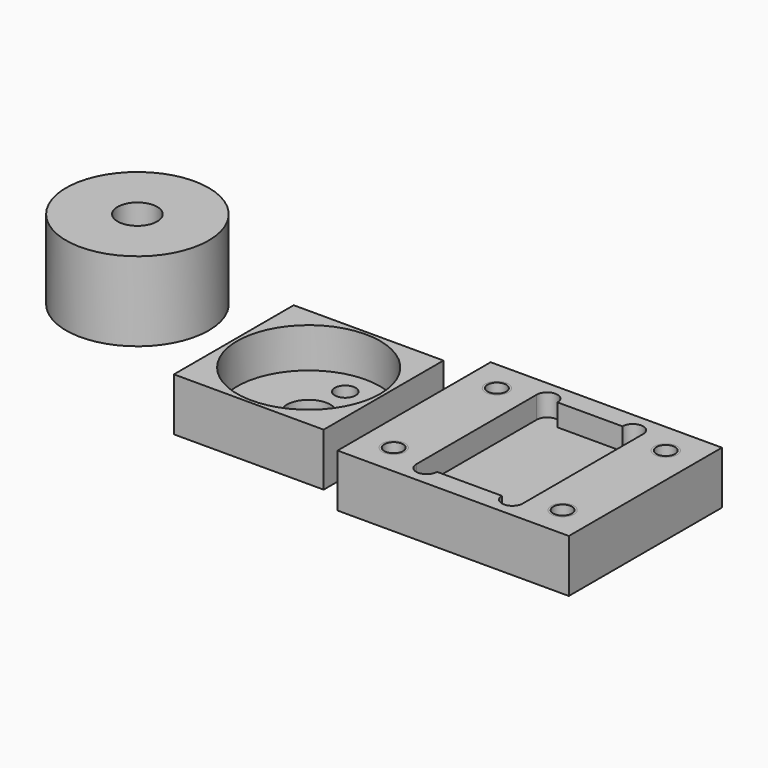
from build123d import *

# Parameters (mm, degrees)
F0_W     = 36
F0_H     = 36
F0_R     = 2.5
F1_DEPTH = 12.7
F2_DEPTH = 9.585
F3_W     = 55.6
F3_H     = 46
F3_R     = 2.75
F3_R_2   = 2.25
F4_DEPTH = 12.7
F5_DEPTH = 11.7
F6_R     = 17.145
F6_R_2   = 4.7625
F7_DEPTH = 19.05
F8_DEPTH = 12.7
F9_DEPTH = 5.3


# Not quite as in the source:
# - a length typed as a fraction of an inch, garbled in the dataset ("3 / 203.2 mm" for 3/8 in), is restored


with BuildPart() as f1:
    # F0 (on Top) → F1 (new body)
    with BuildSketch(Plane.XY):
        Rectangle(F0_W, F0_H)
        with BuildLine():
            ThreePointArc((-17.2, 0), (0, 17.2), (17.2, 0))
            ThreePointArc((17.2, 0), (0, -17.2), (-17.2, 0))
        make_face(mode=Mode.SUBTRACT)
        with BuildLine():
            ThreePointArc((-17.2, 0), (0, -17.2), (17.2, 0))
            ThreePointArc((17.2, 0), (0, 17.2), (-17.2, 0))
        make_face()
        with Locations((0, -10.98125)):
            Circle(F0_R, mode=Mode.SUBTRACT)
        with BuildLine():
            ThreePointArc((5.2625, 0), (0, -5.2625), (-5.2625, 0))
            ThreePointArc((-5.2625, 0), (0, 5.2625), (5.2625, 0))
        make_face(mode=Mode.SUBTRACT)
        with Locations((0, 10.98125)):
            Circle(F0_R, mode=Mode.SUBTRACT)
    extrude(amount=-F1_DEPTH)

    # F0 (on Top) → F2 (cut)
    with BuildSketch(Plane.XY):
        with BuildLine():
            ThreePointArc((-17.2, 0), (0, -17.2), (17.2, 0))
            ThreePointArc((17.2, 0), (0, 17.2), (-17.2, 0))
        make_face()
        with Locations((0, -10.98125)):
            Circle(F0_R, mode=Mode.SUBTRACT)
        with BuildLine():
            ThreePointArc((5.2625, 0), (0, -5.2625), (-5.2625, 0))
            ThreePointArc((-5.2625, 0), (0, 5.2625), (5.2625, 0))
        make_face(mode=Mode.SUBTRACT)
        with Locations((0, 10.98125)):
            Circle(F0_R, mode=Mode.SUBTRACT)
    extrude(amount=-F2_DEPTH, mode=Mode.SUBTRACT)


with BuildPart() as f4:
    # F3 (on Top) → F4 (new body)
    with BuildSketch(Plane.XY):
        with Locations((53.1422479868, 0)):
            Rectangle(F3_W, F3_H)
        with Locations((32.8422479868, -15.5)):
            Circle(F3_R, mode=Mode.SUBTRACT)
        with Locations((73.4422479868, -15.5)):
            Circle(F3_R, mode=Mode.SUBTRACT)
        with BuildLine():
            Line((40.3422479868, -18.1), (40.3422479868, 18.1))
            ThreePointArc((40.3422479868, 18.1), (42.8422479868, 20.6), (45.3422479868, 18.1))
            Line((45.3422479868, 18.1), (60.9422479868, 18.1))
            ThreePointArc((60.9422479868, 18.1), (63.4422479868, 20.6), (65.9422479868, 18.1))
            Line((65.9422479868, 18.1), (65.9422479868, -18.1))
            ThreePointArc((65.9422479868, -18.1), (63.4422479868, -20.6), (60.9422479868, -18.1))
            Line((60.9422479868, -18.1), (45.3422479868, -18.1))
            ThreePointArc((45.3422479868, -18.1), (42.8422479868, -20.6), (40.3422479868, -18.1))
        make_face(mode=Mode.SUBTRACT)
        with Locations((32.8422479868, 15.5)):
            Circle(F3_R, mode=Mode.SUBTRACT)
        with Locations((73.4422479868, 15.5)):
            Circle(F3_R, mode=Mode.SUBTRACT)
        with BuildLine():
            ThreePointArc((45.3422479868, 18.1), (42.8422479868, 20.6), (40.3422479868, 18.1))
            Line((40.3422479868, 18.1), (40.3422479868, -18.1))
            ThreePointArc((40.3422479868, -18.1), (42.8422479868, -20.6), (45.3422479868, -18.1))
            Line((45.3422479868, -18.1), (60.9422479868, -18.1))
            ThreePointArc((60.9422479868, -18.1), (63.4422479868, -20.6), (65.9422479868, -18.1))
            Line((65.9422479868, -18.1), (65.9422479868, 18.1))
            ThreePointArc((65.9422479868, 18.1), (63.4422479868, 20.6), (60.9422479868, 18.1))
            Line((60.9422479868, 18.1), (45.3422479868, 18.1))
        make_face()
        with Locations((32.8422479868, 15.5)):
            Circle(F3_R)
        with Locations((32.8422479868, 15.5)):
            Circle(F3_R_2, mode=Mode.SUBTRACT)
        with Locations((32.8422479868, -15.5)):
            Circle(F3_R)
        with Locations((32.8422479868, -15.5)):
            Circle(F3_R_2, mode=Mode.SUBTRACT)
        with Locations((73.4422479868, -15.5)):
            Circle(F3_R)
        with Locations((73.4422479868, -15.5)):
            Circle(F3_R_2, mode=Mode.SUBTRACT)
        with Locations((73.4422479868, 15.5)):
            Circle(F3_R)
        with Locations((73.4422479868, 15.5)):
            Circle(F3_R_2, mode=Mode.SUBTRACT)
    extrude(amount=-F4_DEPTH)

    # F3 (on Top) → F5 (cut)
    with BuildSketch(Plane.XY):
        with BuildLine():
            ThreePointArc((45.3422479868, 18.1), (42.8422479868, 20.6), (40.3422479868, 18.1))
            Line((40.3422479868, 18.1), (40.3422479868, -18.1))
            ThreePointArc((40.3422479868, -18.1), (42.8422479868, -20.6), (45.3422479868, -18.1))
            Line((45.3422479868, -18.1), (60.9422479868, -18.1))
            ThreePointArc((60.9422479868, -18.1), (63.4422479868, -20.6), (65.9422479868, -18.1))
            Line((65.9422479868, -18.1), (65.9422479868, 18.1))
            ThreePointArc((65.9422479868, 18.1), (63.4422479868, 20.6), (60.9422479868, 18.1))
            Line((60.9422479868, 18.1), (45.3422479868, 18.1))
        make_face()
    extrude(amount=-F5_DEPTH, mode=Mode.SUBTRACT)


with BuildPart() as f7:
    # F6 (on Top) → F7 (new body)
    with BuildSketch(Plane.XY):
        with Locations((-41.1721505225, 0)):
            Circle(F6_R)
        with Locations((-41.1721505225, 0)):
            Circle(F6_R_2, mode=Mode.SUBTRACT)
    extrude(amount=F7_DEPTH)


with BuildPart() as f8:
    # F3 (on Top) → F8 (new body)
    with BuildSketch(Plane.XY):
        with Locations((53.1422479868, 0)):
            Rectangle(F3_W, F3_H)
        with Locations((32.8422479868, -15.5)):
            Circle(F3_R, mode=Mode.SUBTRACT)
        with Locations((73.4422479868, -15.5)):
            Circle(F3_R, mode=Mode.SUBTRACT)
        with BuildLine():
            Line((40.3422479868, -18.1), (40.3422479868, 18.1))
            ThreePointArc((40.3422479868, 18.1), (42.8422479868, 20.6), (45.3422479868, 18.1))
            Line((45.3422479868, 18.1), (60.9422479868, 18.1))
            ThreePointArc((60.9422479868, 18.1), (63.4422479868, 20.6), (65.9422479868, 18.1))
            Line((65.9422479868, 18.1), (65.9422479868, -18.1))
            ThreePointArc((65.9422479868, -18.1), (63.4422479868, -20.6), (60.9422479868, -18.1))
            Line((60.9422479868, -18.1), (45.3422479868, -18.1))
            ThreePointArc((45.3422479868, -18.1), (42.8422479868, -20.6), (40.3422479868, -18.1))
        make_face(mode=Mode.SUBTRACT)
        with Locations((32.8422479868, 15.5)):
            Circle(F3_R, mode=Mode.SUBTRACT)
        with Locations((73.4422479868, 15.5)):
            Circle(F3_R, mode=Mode.SUBTRACT)
        with BuildLine():
            ThreePointArc((45.3422479868, 18.1), (42.8422479868, 20.6), (40.3422479868, 18.1))
            Line((40.3422479868, 18.1), (40.3422479868, -18.1))
            ThreePointArc((40.3422479868, -18.1), (42.8422479868, -20.6), (45.3422479868, -18.1))
            Line((45.3422479868, -18.1), (60.9422479868, -18.1))
            ThreePointArc((60.9422479868, -18.1), (63.4422479868, -20.6), (65.9422479868, -18.1))
            Line((65.9422479868, -18.1), (65.9422479868, 18.1))
            ThreePointArc((65.9422479868, 18.1), (63.4422479868, 20.6), (60.9422479868, 18.1))
            Line((60.9422479868, 18.1), (45.3422479868, 18.1))
        make_face()
    extrude(amount=-F8_DEPTH)

    # F3 (on Top) → F9 (cut)
    with BuildSketch(Plane.XY):
        with BuildLine():
            ThreePointArc((45.3422479868, 18.1), (42.8422479868, 20.6), (40.3422479868, 18.1))
            Line((40.3422479868, 18.1), (40.3422479868, -18.1))
            ThreePointArc((40.3422479868, -18.1), (42.8422479868, -20.6), (45.3422479868, -18.1))
            Line((45.3422479868, -18.1), (60.9422479868, -18.1))
            ThreePointArc((60.9422479868, -18.1), (63.4422479868, -20.6), (65.9422479868, -18.1))
            Line((65.9422479868, -18.1), (65.9422479868, 18.1))
            ThreePointArc((65.9422479868, 18.1), (63.4422479868, 20.6), (60.9422479868, 18.1))
            Line((60.9422479868, 18.1), (45.3422479868, 18.1))
        make_face()
    extrude(amount=-F9_DEPTH, mode=Mode.SUBTRACT)


solid = Compound([f1.part, f4.part, f7.part, f8.part])
